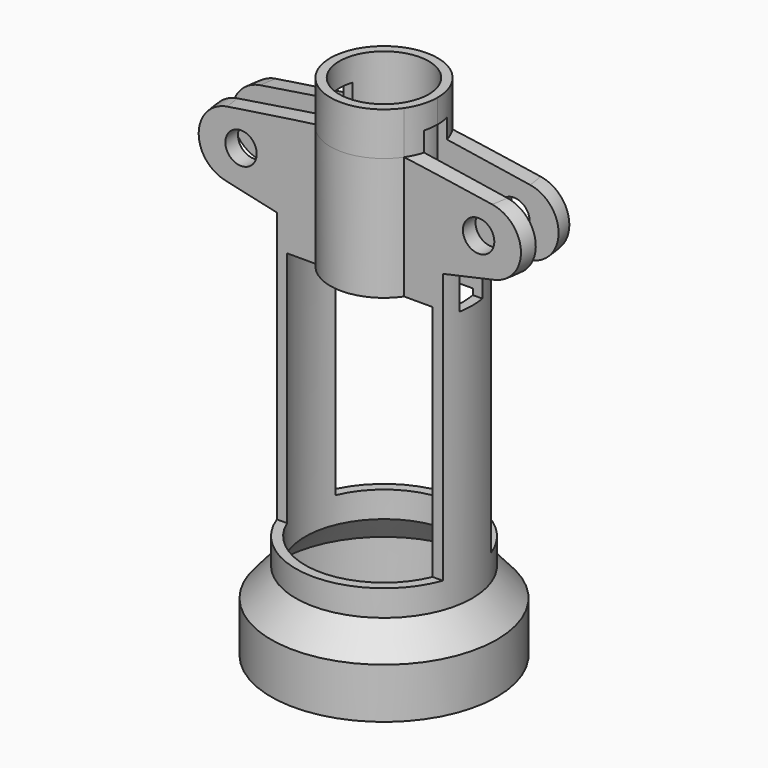
from build123d import *
from build123d import SkipClean  # not in build123d's __all__

# Parameters (mm, degrees)
F3_DEPTH = 68.1
F4_W     = 4.8
F4_H     = 25
F5_DEPTH = 41.80857
F6_R     = 2.65
F7_DEPTH = 25


with BuildPart() as f1:
    # F0 (on Front) → F1 (revolve)
    with BuildSketch(Plane.XZ):
        with BuildLine():
            Line((17.45, 8.5), (17.45, 0))
            Line((17.45, 0), (19.05, 0))
            Line((19.05, 0), (19.05, 8.5))
            Line((19.05, 8.5), (14.9, 13.3))
            Line((14.9, 13.3), (14.9, 63.3))
            Line((14.9, 63.3), (23.2882495839, 65.2334026039))
            ThreePointArc((23.2882495839, 65.2334026039), (27.6657550526, 70.9379230726), (22.8977616622, 76.3203339576))
            Line((22.8977616622, 76.3203339576), (9.05, 78.5))
            Line((9.05, 78.5), (9.05, 85.8))
            Line((9.05, 85.8), (7.55, 85.8))
            Line((7.55, 85.8), (7.55, 57.8))
            Line((7.55, 57.8), (13.3, 57.8))
            Line((13.3, 57.8), (13.3, 13.3))
            Line((13.3, 13.3), (17.45, 8.5))
        make_face()
    revolve(axis=Axis((0, 0, 43.5625389218), (0, 0, 1)))

    # F2 (on face) → F3 (cut)
    with BuildSketch(Plane.XY.offset(85.8)):
        with BuildLine():
            ThreePointArc((7.4761286773, -5.1), (0, -9.05), (-7.4761286773, -5.1))
            Line((-7.4761286773, -5.1), (-33.3200879395, -5.1))
            Line((-33.3200879395, -5.1), (-33.3200879395, -32.3637121379))
            Line((-33.3200879395, -32.3637121379), (33.8455328711, -32.3637121379))
            Line((33.8455328711, -32.3637121379), (33.8455328711, -5.1))
            Line((33.8455328711, -5.1), (7.4761286773, -5.1))
        make_face()
        with BuildLine():
            Line((7.4761286773, 5.1), (33.8455328711, 5.1))
            Line((33.8455328711, 5.1), (33.8455328711, 32.3637121379))
            Line((33.8455328711, 32.3637121379), (-33.3200879395, 32.3637121379))
            Line((-33.3200879395, 32.3637121379), (-33.3200879395, 5.1))
            Line((-33.3200879395, 5.1), (-7.4761286773, 5.1))
            ThreePointArc((-7.4761286773, 5.1), (0, 9.05), (7.4761286773, 5.1))
        make_face()
    with SkipClean():  # cleaning this boolean's faces spoils the solid; the shape is the same uncleaned
        extrude(amount=-F3_DEPTH, mode=Mode.SUBTRACT)

    # F4 (on Right) → F5 (cut, symmetric)
    with BuildSketch(Plane.YZ):
        with Locations((-0.0327096786, 69.3)):
            Rectangle(F4_W, F4_H)
    extrude(amount=F5_DEPTH, both=True, mode=Mode.SUBTRACT)

    # F6 (on face) → F7 (cut)
    with BuildSketch(Plane(origin=(0, 5.1, 0), x_dir=(-1, 0, 0), z_dir=(0, 1, 0))):
        with Locations((-20.0461286773, 70.9)):
            Circle(F6_R)
        with Locations((20.0461286773, 70.9)):
            Circle(F6_R)
    extrude(amount=-F7_DEPTH, mode=Mode.SUBTRACT)


solid = f1.part
